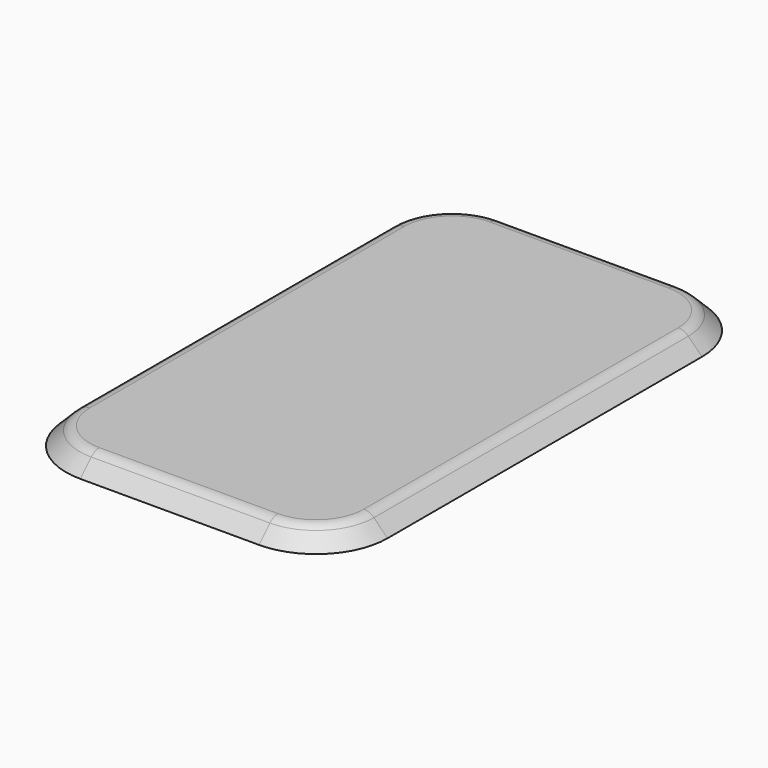
from build123d import *

# Parameters (mm, degrees)
F1_DEPTH = 5
F2_SIZE  = 4.99999
F3_R     = 4


# Not quite as in the source:
# - a fillet or chamfer is up to 0.001 mm smaller than in the source, because OpenCascade refuses the exact size


with BuildPart() as f1:
    # F0 (on Top) → F1 (new body)
    with BuildSketch(Plane.XY):
        with BuildLine():
            Line((25, 75), (-25, 75))
            ThreePointArc((-25, 75), (-39.1421356237, 69.1421356237), (-45, 55))
            Line((-45, 55), (-45, -55))
            ThreePointArc((-45, -55), (-39.1421356237, -69.1421356237), (-25, -75))
            Line((-25, -75), (25, -75))
            ThreePointArc((25, -75), (39.1421356237, -69.1421356237), (45, -55))
            Line((45, -55), (45, 55))
            ThreePointArc((45, 55), (39.1421356237, 69.1421356237), (25, 75))
        make_face()
    extrude(amount=F1_DEPTH)

    # F2 (size 5 in the source; OpenCascade refuses exactly that, so slightly less here)
    f2_edges = [f1.edges().sort_by_distance(p)[0] for p in [
        (-39.142136, -69.142136, 5),
        (0, -75, 5),
        (39.142136, -69.142136, 5),
        (45, 0, 5),
        (39.142136, 69.142136, 5),
        (0, 75, 5),
        (-39.142136, 69.142136, 5),
        (-45, 0, 5),
    ]]
    chamfer(f2_edges, length=F2_SIZE)

    # F3
    f3_edges = [f1.edges().sort_by_distance(p)[0] for p in [
        (-35.606609, -65.606609, 5),
        (-40.00001, 0, 5),
        (0, -70.00001, 5),
        (-35.606609, 65.606609, 5),
        (35.606609, -65.606609, 5),
        (0, 70.00001, 5),
        (40.00001, 0, 5),
        (35.606609, 65.606609, 5),
    ]]
    fillet(f3_edges, radius=F3_R)


solid = f1.part
